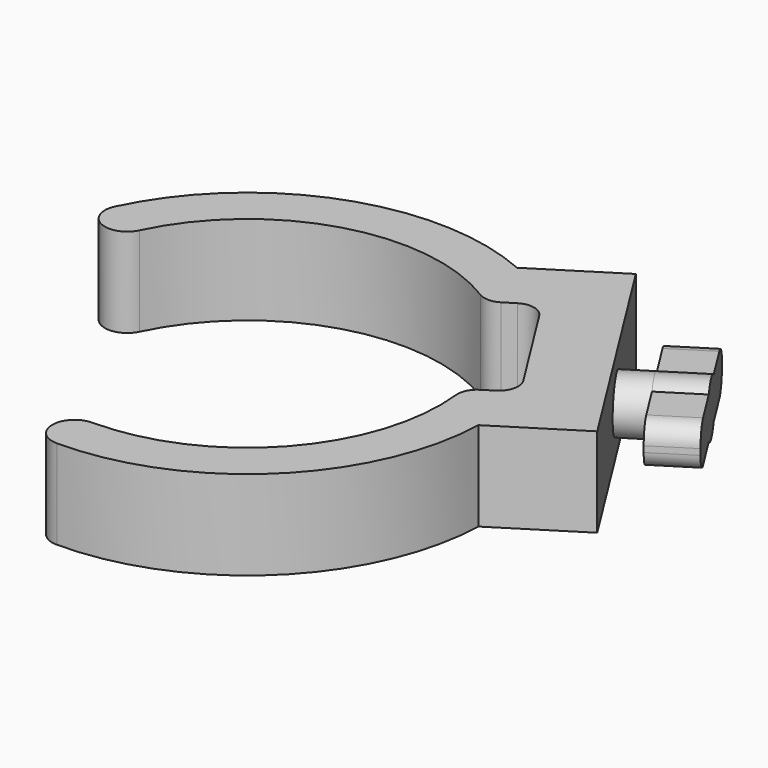
from build123d import *

# Parameters (mm, degrees)
F1_DEPTH = 6
F2_R     = 1.8
F3_DEPTH = 2
F5_DEPTH = 3
F6_R     = 1.2
F8_DEPTH = 6.1
F9_R     = 1.3


# Not quite as in the source:
# - a feature names something its author has since deleted; it is built from what else it names


with BuildPart() as f1:
    # F0 (on Top) → F1 (new body)
    with BuildSketch(Plane.XY):
        with BuildLine():
            ThreePointArc((11, 6.9282032303), (11.3812706231, -6.2822511095), (0, -13))
            ThreePointArc((0, -13), (-1.5000000067, -14.4999999933), (-1.34e-08, -16))
            ThreePointArc((-1.34e-08, -16), (11.1120589721, -11.5118263277), (15.9900116293, -0.5652681616))
            Line((15.9900116293, -0.5652681616), (15.7964483902, -0.6871813851))
            Line((15.7964483902, -0.6871813851), (11, 6.9282032303))
        make_face()
        with BuildLine():
            ThreePointArc((-11.7246516205, 5.6153846154), (-0.7497687455, 12.9783607142), (11, 6.9282032303))
            Line((11, 6.9282032303), (6.2035516098, 14.5435878457))
            Line((6.2035516098, 14.5435878457), (6.3971148489, 14.6655010692))
            ThreePointArc((6.3971148489, 14.6655010692), (-5.582589802, 14.9944886909), (-14.4303404061, 6.9112427076))
            ThreePointArc((-14.4303404061, 6.9112427076), (-13.7254250594, 4.9104692687), (-11.7246516205, 5.6153846154))
        make_face()
        with BuildLine():
            Line((6.2035516098, 14.5435878457), (11, 6.9282032303))
            Line((11, 6.9282032303), (15.7964483902, -0.6871813851))
            Line((15.7964483902, -0.6871813851), (15.9900116293, -0.5652681616))
            ThreePointArc((15.9900116293, -0.5652681616), (13.5384615385, 8.5270193603), (6.3971148489, 14.6655010692))
            Line((6.3971148489, 14.6655010692), (6.2035516098, 14.5435878457))
        make_face()
        with BuildLine():
            ThreePointArc((6.3971148489, 14.6655010692), (13.5384615385, 8.5270193603), (15.9900116293, -0.5652681616))
            Line((15.9900116293, -0.5652681616), (21.2964483902, 2.77692023))
            Line((21.2964483902, 2.77692023), (11.7035516098, 18.0076894608))
            Line((11.7035516098, 18.0076894608), (6.3971148489, 14.6655010692))
        make_face()
    extrude(amount=F1_DEPTH)

    # F2 (on face) → F3 (join)
    with BuildSketch(Plane(origin=(16.5, 10.3923048454, 0), x_dir=(-0.53293871, 0.8461538462, 0), z_dir=(0.8461538462, 0.53293871, 0))):
        with Locations((0, 3)):
            Circle(F2_R)
    extrude(amount=F3_DEPTH)

    # F4 (on face) → F5 (join)
    with BuildSketch(Plane(origin=(18.1923076923, 11.4581822655, 0), x_dir=(-0.53293871, 0.8461538462, 0), z_dir=(0.8461538462, 0.53293871, 0))):
        with BuildLine():
            Line((-1.1313708499, 4.4), (1.1313708499, 4.4))
            ThreePointArc((1.1313708499, 4.4), (0, 4.8), (-1.1313708499, 4.4))
        make_face()
        with BuildLine():
            Line((-1.1313708499, 1.6), (1.1313708499, 1.6))
            ThreePointArc((1.1313708499, 1.6), (1.6242640687, 2.2242640687), (1.8, 3))
            ThreePointArc((1.8, 3), (1.6242640687, 3.7757359313), (1.1313708499, 4.4))
            Line((1.1313708499, 4.4), (-1.1313708499, 4.4))
            ThreePointArc((-1.1313708499, 4.4), (-1.8, 3), (-1.1313708499, 1.6))
        make_face()
        with BuildLine():
            Line((1.1313708499, 1.6), (5, 1.6))
            Line((5, 1.6), (5, 4.4))
            Line((5, 4.4), (1.1313708499, 4.4))
            ThreePointArc((1.1313708499, 4.4), (1.6242640687, 3.7757359313), (1.8, 3))
            ThreePointArc((1.8, 3), (1.6242640687, 2.2242640687), (1.1313708499, 1.6))
        make_face()
        with BuildLine():
            Line((-5, 1.6), (-1.1313708499, 1.6))
            ThreePointArc((-1.1313708499, 1.6), (-1.8, 3), (-1.1313708499, 4.4))
            Line((-1.1313708499, 4.4), (-5, 4.4))
            Line((-5, 4.4), (-5, 1.6))
        make_face()
        with BuildLine():
            ThreePointArc((-1.1313708499, 1.6), (0, 1.2), (1.1313708499, 1.6))
            Line((1.1313708499, 1.6), (-1.1313708499, 1.6))
        make_face()
    extrude(amount=F5_DEPTH)

    # F6
    f6_edges = [f1.edges().sort_by_distance(p)[0] for p in [
        (22.126232, 8.026821, 4.4),
        (22.126232, 8.026821, 1.6),
        (16.796845, 16.48836, 4.4),
        (16.796845, 16.48836, 1.6),
    ]]
    fillet(f6_edges, radius=F6_R)

    # F7 (on face) → F8 (cut)
    with BuildSketch(Plane.XY.offset(6)):
        with BuildLine():
            ThreePointArc((7.4891526037, 10.626033751), (9.4276549916, 8.9509396914), (11, 6.9282032303))
            Line((11, 6.9282032303), (12.6923076923, 7.9940806503))
            Line((12.6923076923, 7.9940806503), (10.0276141422, 12.2248498811))
            Line((10.0276141422, 12.2248498811), (7.4891526037, 10.626033751))
        make_face()
        with BuildLine():
            Line((12.6923076923, 7.9940806503), (11, 6.9282032303))
            ThreePointArc((11, 6.9282032303), (12.1451198736, 4.6363847183), (12.818539704, 2.1644952895))
            Line((12.818539704, 2.1644952895), (15.3570012424, 3.7633114195))
            Line((15.3570012424, 3.7633114195), (12.6923076923, 7.9940806503))
        make_face()
    extrude(amount=-F8_DEPTH, mode=Mode.SUBTRACT)

    # F9
    f9_edges = [f1.edges().sort_by_distance(p)[0] for p in [
        (7.489153, 10.626034, 3),
        (10.027614, 12.22485, 3),
        (12.81854, 2.164495, 3),
        (15.357001, 3.763311, 3),
    ]]
    fillet(f9_edges, radius=F9_R)


solid = f1.part
